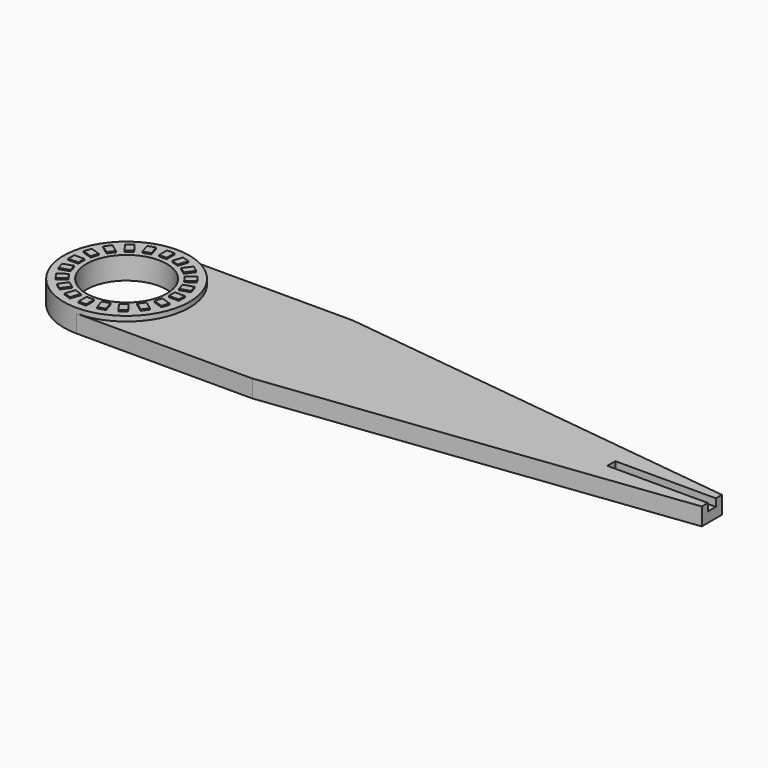
from build123d import *

# Parameters (mm, degrees)
F0_R         = 8
F1_DEPTH     = 3.5
F2_R         = 12.5
F2_R_2       = 8
F3_DEPTH     = 1
F4_W         = 1.5
F4_H         = 2
F4_W_2       = 2
F4_H_2       = 1.5
F5_DEPTH     = 0.25
F6_W         = 20
F6_H         = 2
F7_DEPTH     = 1.5
F9_TEXT_SIZE = 15.5695032355
F10_DEPTH    = 1.5


# Not quite as in the source:
# - Text() gives the source's letters only with a copy of the font that has no kerning and outlines rounded to 1/6400 em; it was checked with that copy


with BuildPart() as f1:
    # F0 (on Top) → F1 (new body)
    with BuildSketch(Plane.XY):
        with BuildLine():
            Line((35, 12.5), (0, 12.5))
            ThreePointArc((0, 12.5), (-12.5, 0), (0, -12.5))
            Line((0, -12.5), (35, -12.5))
            Line((35, -12.5), (116.3887844346, -2.5067138408))
            Line((116.3887844346, -2.5067138408), (116.3887844346, 2.5067138408))
            Line((116.3887844346, 2.5067138408), (35, 12.5))
        make_face()
        Circle(F0_R, mode=Mode.SUBTRACT)
    extrude(amount=F1_DEPTH)

    # F2 (on face) → F3 (join)
    with BuildSketch(Plane.XY.offset(3.5)):
        Circle(F2_R)
        Circle(F2_R_2, mode=Mode.SUBTRACT)
    extrude(amount=F3_DEPTH)

    # F4 (on face) → F5 (join)
    with BuildSketch(Plane.XY.offset(4.5)):
        with Locations((0, 10)):
            Rectangle(F4_W, F4_H)
        Polygon((-2.6858945509, 10.693384425), (-4.1124793253, 10.2298589335), (-3.4944453366, 8.3277459009), (-2.0678605622, 8.7912713924), align=None)
        Polygon((-5.8588750294, 9.3400258773), (-7.072400521, 8.4583479989), (-5.8968300164, 6.8403140102), (-4.6833045249, 7.7219918886), align=None)
        Polygon((-8.4583479989, 7.072400521), (-9.3400258773, 5.8588750294), (-7.7219918886, 4.6833045249), (-6.8403140102, 5.8968300164), align=None)
        Polygon((-10.2298589335, 4.1124793253), (-10.693384425, 2.6858945509), (-8.7912713924, 2.0678605622), (-8.3277459009, 3.4944453366), align=None)
        with Locations((-10, 0)):
            Rectangle(F4_W_2, F4_H_2)
        Polygon((-10.693384425, -2.6858945509), (-10.2298589335, -4.1124793253), (-8.3277459009, -3.4944453366), (-8.7912713924, -2.0678605622), align=None)
        Polygon((-9.3400258773, -5.8588750294), (-8.4583479989, -7.072400521), (-6.8403140102, -5.8968300164), (-7.7219918886, -4.6833045249), align=None)
        Polygon((-7.072400521, -8.4583479989), (-5.8588750294, -9.3400258773), (-4.6833045249, -7.7219918886), (-5.8968300164, -6.8403140102), align=None)
        Polygon((-4.1124793253, -10.2298589335), (-2.6858945509, -10.693384425), (-2.0678605622, -8.7912713924), (-3.4944453366, -8.3277459009), align=None)
        with Locations((0, -10)):
            Rectangle(F4_W, F4_H)
        Polygon((2.6858945509, -10.693384425), (4.1124793253, -10.2298589335), (3.4944453366, -8.3277459009), (2.0678605622, -8.7912713924), align=None)
        Polygon((5.8588750294, -9.3400258773), (7.072400521, -8.4583479989), (5.8968300164, -6.8403140102), (4.6833045249, -7.7219918886), align=None)
        Polygon((8.4583479989, -7.072400521), (9.3400258773, -5.8588750294), (7.7219918886, -4.6833045249), (6.8403140102, -5.8968300164), align=None)
        Polygon((10.2298589335, -4.1124793253), (10.693384425, -2.6858945509), (8.7912713924, -2.0678605622), (8.3277459009, -3.4944453366), align=None)
        with Locations((10, 0)):
            Rectangle(F4_W_2, F4_H_2)
        Polygon((10.693384425, 2.6858945509), (10.2298589335, 4.1124793253), (8.3277459009, 3.4944453366), (8.7912713924, 2.0678605622), align=None)
        Polygon((9.3400258773, 5.8588750294), (8.4583479989, 7.072400521), (6.8403140102, 5.8968300164), (7.7219918886, 4.6833045249), align=None)
        Polygon((7.072400521, 8.4583479989), (5.8588750294, 9.3400258773), (4.6833045249, 7.7219918886), (5.8968300164, 6.8403140102), align=None)
        Polygon((4.1124793253, 10.2298589335), (2.6858945509, 10.693384425), (2.0678605622, 8.7912713924), (3.4944453366, 8.3277459009), align=None)
    extrude(amount=F5_DEPTH)

    # F6 (on face) → F7 (cut)
    with BuildSketch(Plane.XY.offset(3.5)):
        with Locations((106.3887844346, 0.0067138408)):
            Rectangle(F6_W, F6_H)
    extrude(amount=-F7_DEPTH, mode=Mode.SUBTRACT)

    # F9 (on face) → F10 (cut)
    with BuildSketch(Plane(origin=(0, 0, 0), x_dir=(1, 0, 0), z_dir=(0, 0, -1))):
        with Locations((12, -5.6050211648)):
            Text('Ronnie', F9_TEXT_SIZE, font='Open Sans', text_align=(TextAlign.LEFT, TextAlign.BOTTOM))
    extrude(amount=-F10_DEPTH, mode=Mode.SUBTRACT)


solid = f1.part
